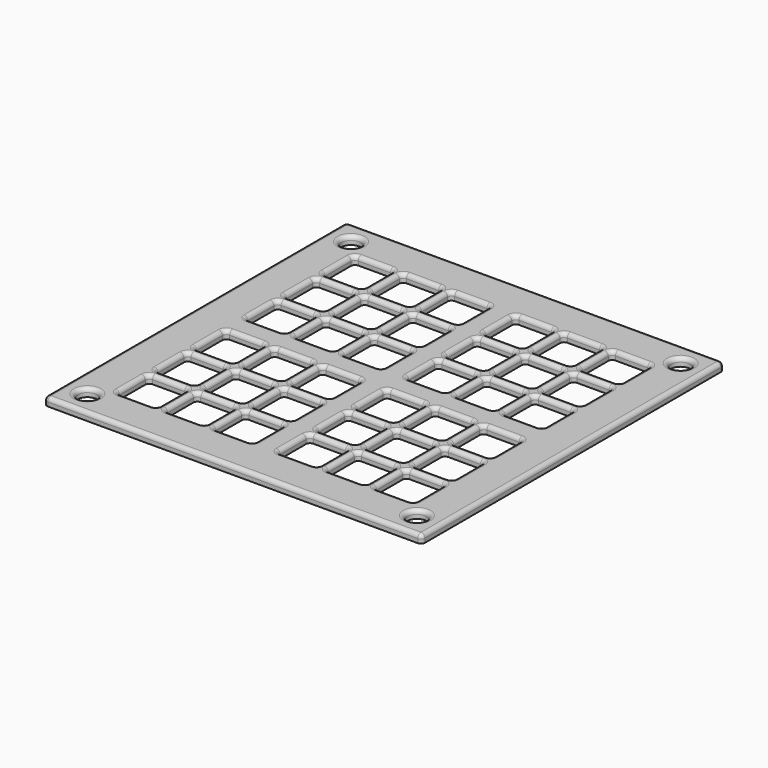
from build123d import *

# Parameters (mm, degrees)
F0_W     = 119.38
F0_H     = 119.38
F0_R     = 3.048
F1_DEPTH = 2.54
F2_R     = 1.26999


# Not quite as in the source:
# - a fillet or chamfer is up to 0.001 mm smaller than in the source, because OpenCascade refuses the exact size


with BuildPart() as f1:
    # F0 (on Top) → F1 (new body)
    with BuildSketch(Plane.XY):
        Rectangle(F0_W, F0_H)
        with Locations((-52.07, -52.07)):
            Circle(F0_R, mode=Mode.SUBTRACT)
        with BuildLine():
            Line((-46.99, -45.72), (-46.99, -35.56))
            ThreePointArc((-46.99, -35.56), (-46.6180256121, -34.6619743879), (-45.72, -34.29))
            Line((-45.72, -34.29), (-35.56, -34.29))
            ThreePointArc((-35.56, -34.29), (-34.6619743879, -34.6619743879), (-34.29, -35.56))
            Line((-34.29, -35.56), (-34.29, -45.72))
            ThreePointArc((-34.29, -45.72), (-34.6619743879, -46.6180256121), (-35.56, -46.99))
            Line((-35.56, -46.99), (-45.72, -46.99))
            ThreePointArc((-45.72, -46.99), (-46.6180256121, -46.6180256121), (-46.99, -45.72))
        make_face(mode=Mode.SUBTRACT)
        with BuildLine():
            Line((-20.32, -46.99), (-30.48, -46.99))
            ThreePointArc((-30.48, -46.99), (-31.3780256121, -46.6180256121), (-31.75, -45.72))
            Line((-31.75, -45.72), (-31.75, -35.56))
            ThreePointArc((-31.75, -35.56), (-31.3780256121, -34.6619743879), (-30.48, -34.29))
            Line((-30.48, -34.29), (-20.32, -34.29))
            ThreePointArc((-20.32, -34.29), (-19.4219743879, -34.6619743879), (-19.05, -35.56))
            Line((-19.05, -35.56), (-19.05, -45.72))
            ThreePointArc((-19.05, -45.72), (-19.4219743879, -46.6180256121), (-20.32, -46.99))
        make_face(mode=Mode.SUBTRACT)
        with BuildLine():
            Line((-15.24, -34.29), (-5.08, -34.29))
            ThreePointArc((-5.08, -34.29), (-4.1819743879, -34.6619743879), (-3.81, -35.56))
            Line((-3.81, -35.56), (-3.81, -45.72))
            ThreePointArc((-3.81, -45.72), (-4.1819743879, -46.6180256121), (-5.08, -46.99))
            Line((-5.08, -46.99), (-15.24, -46.99))
            ThreePointArc((-15.24, -46.99), (-16.1380256121, -46.6180256121), (-16.51, -45.72))
            Line((-16.51, -45.72), (-16.51, -35.56))
            ThreePointArc((-16.51, -35.56), (-16.1380256121, -34.6619743879), (-15.24, -34.29))
        make_face(mode=Mode.SUBTRACT)
        with BuildLine():
            Line((-34.29, -20.32), (-34.29, -30.48))
            ThreePointArc((-34.29, -30.48), (-34.6619743879, -31.3780256121), (-35.56, -31.75))
            Line((-35.56, -31.75), (-45.72, -31.75))
            ThreePointArc((-45.72, -31.75), (-46.6180256121, -31.3780256121), (-46.99, -30.48))
            Line((-46.99, -30.48), (-46.99, -20.32))
            ThreePointArc((-46.99, -20.32), (-46.6180256121, -19.4219743879), (-45.72, -19.05))
            Line((-45.72, -19.05), (-35.56, -19.05))
            ThreePointArc((-35.56, -19.05), (-34.6619743879, -19.4219743879), (-34.29, -20.32))
        make_face(mode=Mode.SUBTRACT)
        with BuildLine():
            Line((-45.72, -3.81), (-35.56, -3.81))
            ThreePointArc((-35.56, -3.81), (-34.6619743879, -4.1819743879), (-34.29, -5.08))
            Line((-34.29, -5.08), (-34.29, -15.24))
            ThreePointArc((-34.29, -15.24), (-34.6619743879, -16.1380256121), (-35.56, -16.51))
            Line((-35.56, -16.51), (-45.72, -16.51))
            ThreePointArc((-45.72, -16.51), (-46.6180256121, -16.1380256121), (-46.99, -15.24))
            Line((-46.99, -15.24), (-46.99, -5.08))
            ThreePointArc((-46.99, -5.08), (-46.6180256121, -4.1819743879), (-45.72, -3.81))
        make_face(mode=Mode.SUBTRACT)
        with BuildLine():
            Line((-30.48, -19.05), (-20.32, -19.05))
            ThreePointArc((-20.32, -19.05), (-19.4219743879, -19.4219743879), (-19.05, -20.32))
            Line((-19.05, -20.32), (-19.05, -30.48))
            ThreePointArc((-19.05, -30.48), (-19.4219743879, -31.3780256121), (-20.32, -31.75))
            Line((-20.32, -31.75), (-30.48, -31.75))
            ThreePointArc((-30.48, -31.75), (-31.3780256121, -31.3780256121), (-31.75, -30.48))
            Line((-31.75, -30.48), (-31.75, -20.32))
            ThreePointArc((-31.75, -20.32), (-31.3780256121, -19.4219743879), (-30.48, -19.05))
        make_face(mode=Mode.SUBTRACT)
        with BuildLine():
            Line((-5.08, -31.75), (-15.24, -31.75))
            ThreePointArc((-15.24, -31.75), (-16.1380256121, -31.3780256121), (-16.51, -30.48))
            Line((-16.51, -30.48), (-16.51, -20.32))
            ThreePointArc((-16.51, -20.32), (-16.1380256121, -19.4219743879), (-15.24, -19.05))
            Line((-15.24, -19.05), (-5.08, -19.05))
            ThreePointArc((-5.08, -19.05), (-4.1819743879, -19.4219743879), (-3.81, -20.32))
            Line((-3.81, -20.32), (-3.81, -30.48))
            ThreePointArc((-3.81, -30.48), (-4.1819743879, -31.3780256121), (-5.08, -31.75))
        make_face(mode=Mode.SUBTRACT)
        with BuildLine():
            Line((-31.75, -15.24), (-31.75, -5.08))
            ThreePointArc((-31.75, -5.08), (-31.3780256121, -4.1819743879), (-30.48, -3.81))
            Line((-30.48, -3.81), (-20.32, -3.81))
            ThreePointArc((-20.32, -3.81), (-19.4219743879, -4.1819743879), (-19.05, -5.08))
            Line((-19.05, -5.08), (-19.05, -15.24))
            ThreePointArc((-19.05, -15.24), (-19.4219743879, -16.1380256121), (-20.32, -16.51))
            Line((-20.32, -16.51), (-30.48, -16.51))
            ThreePointArc((-30.48, -16.51), (-31.3780256121, -16.1380256121), (-31.75, -15.24))
        make_face(mode=Mode.SUBTRACT)
        with BuildLine():
            Line((-15.24, -3.81), (-5.08, -3.81))
            ThreePointArc((-5.08, -3.81), (-4.1819743879, -4.1819743879), (-3.81, -5.08))
            Line((-3.81, -5.08), (-3.81, -15.24))
            ThreePointArc((-3.81, -15.24), (-4.1819743879, -16.1380256121), (-5.08, -16.51))
            Line((-5.08, -16.51), (-15.24, -16.51))
            ThreePointArc((-15.24, -16.51), (-16.1380256121, -16.1380256121), (-16.51, -15.24))
            Line((-16.51, -15.24), (-16.51, -5.08))
            ThreePointArc((-16.51, -5.08), (-16.1380256121, -4.1819743879), (-15.24, -3.81))
        make_face(mode=Mode.SUBTRACT)
        with BuildLine():
            Line((3.81, -45.72), (3.81, -35.56))
            ThreePointArc((3.81, -35.56), (4.1819743879, -34.6619743879), (5.08, -34.29))
            Line((5.08, -34.29), (15.24, -34.29))
            ThreePointArc((15.24, -34.29), (16.1380256121, -34.6619743879), (16.51, -35.56))
            Line((16.51, -35.56), (16.51, -45.72))
            ThreePointArc((16.51, -45.72), (16.1380256121, -46.6180256121), (15.24, -46.99))
            Line((15.24, -46.99), (5.08, -46.99))
            ThreePointArc((5.08, -46.99), (4.1819743879, -46.6180256121), (3.81, -45.72))
        make_face(mode=Mode.SUBTRACT)
        with BuildLine():
            Line((19.05, -45.72), (19.05, -35.56))
            ThreePointArc((19.05, -35.56), (19.4219743879, -34.6619743879), (20.32, -34.29))
            Line((20.32, -34.29), (30.48, -34.29))
            ThreePointArc((30.48, -34.29), (31.3780256121, -34.6619743879), (31.75, -35.56))
            Line((31.75, -35.56), (31.75, -45.72))
            ThreePointArc((31.75, -45.72), (31.3780256121, -46.6180256121), (30.48, -46.99))
            Line((30.48, -46.99), (20.32, -46.99))
            ThreePointArc((20.32, -46.99), (19.4219743879, -46.6180256121), (19.05, -45.72))
        make_face(mode=Mode.SUBTRACT)
        with Locations((52.07, -52.07)):
            Circle(F0_R, mode=Mode.SUBTRACT)
        with BuildLine():
            ThreePointArc((34.29, -35.56), (34.6619743879, -34.6619743879), (35.56, -34.29))
            Line((35.56, -34.29), (45.72, -34.29))
            ThreePointArc((45.72, -34.29), (46.6180256121, -34.6619743879), (46.99, -35.56))
            Line((46.99, -35.56), (46.99, -45.72))
            ThreePointArc((46.99, -45.72), (46.6180256121, -46.6180256121), (45.72, -46.99))
            Line((45.72, -46.99), (35.56, -46.99))
            ThreePointArc((35.56, -46.99), (34.6619743879, -46.6180256121), (34.29, -45.72))
            Line((34.29, -45.72), (34.29, -35.56))
        make_face(mode=Mode.SUBTRACT)
        with BuildLine():
            Line((3.81, -30.48), (3.81, -20.32))
            ThreePointArc((3.81, -20.32), (4.1819743879, -19.4219743879), (5.08, -19.05))
            Line((5.08, -19.05), (15.24, -19.05))
            ThreePointArc((15.24, -19.05), (16.1380256121, -19.4219743879), (16.51, -20.32))
            Line((16.51, -20.32), (16.51, -30.48))
            ThreePointArc((16.51, -30.48), (16.1380256121, -31.3780256121), (15.24, -31.75))
            Line((15.24, -31.75), (5.08, -31.75))
            ThreePointArc((5.08, -31.75), (4.1819743879, -31.3780256121), (3.81, -30.48))
        make_face(mode=Mode.SUBTRACT)
        with BuildLine():
            Line((19.05, -30.48), (19.05, -20.32))
            ThreePointArc((19.05, -20.32), (19.4219743879, -19.4219743879), (20.32, -19.05))
            Line((20.32, -19.05), (30.48, -19.05))
            ThreePointArc((30.48, -19.05), (31.3780256121, -19.4219743879), (31.75, -20.32))
            Line((31.75, -20.32), (31.75, -30.48))
            ThreePointArc((31.75, -30.48), (31.3780256121, -31.3780256121), (30.48, -31.75))
            Line((30.48, -31.75), (20.32, -31.75))
            ThreePointArc((20.32, -31.75), (19.4219743879, -31.3780256121), (19.05, -30.48))
        make_face(mode=Mode.SUBTRACT)
        with BuildLine():
            Line((3.81, -15.24), (3.81, -5.08))
            ThreePointArc((3.81, -5.08), (4.1819743879, -4.1819743879), (5.08, -3.81))
            Line((5.08, -3.81), (15.24, -3.81))
            ThreePointArc((15.24, -3.81), (16.1380256121, -4.1819743879), (16.51, -5.08))
            Line((16.51, -5.08), (16.51, -15.24))
            ThreePointArc((16.51, -15.24), (16.1380256121, -16.1380256121), (15.24, -16.51))
            Line((15.24, -16.51), (5.08, -16.51))
            ThreePointArc((5.08, -16.51), (4.1819743879, -16.1380256121), (3.81, -15.24))
        make_face(mode=Mode.SUBTRACT)
        with BuildLine():
            Line((19.05, -15.24), (19.05, -5.08))
            ThreePointArc((19.05, -5.08), (19.4219743879, -4.1819743879), (20.32, -3.81))
            Line((20.32, -3.81), (30.48, -3.81))
            ThreePointArc((30.48, -3.81), (31.3780256121, -4.1819743879), (31.75, -5.08))
            Line((31.75, -5.08), (31.75, -15.24))
            ThreePointArc((31.75, -15.24), (31.3780256121, -16.1380256121), (30.48, -16.51))
            Line((30.48, -16.51), (20.32, -16.51))
            ThreePointArc((20.32, -16.51), (19.4219743879, -16.1380256121), (19.05, -15.24))
        make_face(mode=Mode.SUBTRACT)
        with BuildLine():
            Line((34.29, -30.48), (34.29, -20.32))
            ThreePointArc((34.29, -20.32), (34.6619743879, -19.4219743879), (35.56, -19.05))
            Line((35.56, -19.05), (45.72, -19.05))
            ThreePointArc((45.72, -19.05), (46.6180256121, -19.4219743879), (46.99, -20.32))
            Line((46.99, -20.32), (46.99, -30.48))
            ThreePointArc((46.99, -30.48), (46.6180256121, -31.3780256121), (45.72, -31.75))
            Line((45.72, -31.75), (35.56, -31.75))
            ThreePointArc((35.56, -31.75), (34.6619743879, -31.3780256121), (34.29, -30.48))
        make_face(mode=Mode.SUBTRACT)
        with BuildLine():
            Line((34.29, -15.24), (34.29, -5.08))
            ThreePointArc((34.29, -5.08), (34.6619743879, -4.1819743879), (35.56, -3.81))
            Line((35.56, -3.81), (45.72, -3.81))
            ThreePointArc((45.72, -3.81), (46.6180256121, -4.1819743879), (46.99, -5.08))
            Line((46.99, -5.08), (46.99, -15.24))
            ThreePointArc((46.99, -15.24), (46.6180256121, -16.1380256121), (45.72, -16.51))
            Line((45.72, -16.51), (35.56, -16.51))
            ThreePointArc((35.56, -16.51), (34.6619743879, -16.1380256121), (34.29, -15.24))
        make_face(mode=Mode.SUBTRACT)
        with BuildLine():
            ThreePointArc((-46.99, 15.24), (-46.6180256121, 16.1380256121), (-45.72, 16.51))
            Line((-45.72, 16.51), (-35.56, 16.51))
            ThreePointArc((-35.56, 16.51), (-34.6619743879, 16.1380256121), (-34.29, 15.24))
            Line((-34.29, 15.24), (-34.29, 5.08))
            ThreePointArc((-34.29, 5.08), (-34.6619743879, 4.1819743879), (-35.56, 3.81))
            Line((-35.56, 3.81), (-45.72, 3.81))
            ThreePointArc((-45.72, 3.81), (-46.6180256121, 4.1819743879), (-46.99, 5.08))
            Line((-46.99, 5.08), (-46.99, 15.24))
        make_face(mode=Mode.SUBTRACT)
        with BuildLine():
            ThreePointArc((-34.29, 20.32), (-34.6619743879, 19.4219743879), (-35.56, 19.05))
            Line((-35.56, 19.05), (-45.72, 19.05))
            ThreePointArc((-45.72, 19.05), (-46.6180256121, 19.4219743879), (-46.99, 20.32))
            Line((-46.99, 20.32), (-46.99, 30.48))
            ThreePointArc((-46.99, 30.48), (-46.6180256121, 31.3780256121), (-45.72, 31.75))
            Line((-45.72, 31.75), (-35.56, 31.75))
            ThreePointArc((-35.56, 31.75), (-34.6619743879, 31.3780256121), (-34.29, 30.48))
            Line((-34.29, 30.48), (-34.29, 20.32))
        make_face(mode=Mode.SUBTRACT)
        with BuildLine():
            ThreePointArc((-30.48, 3.81), (-31.3780256121, 4.1819743879), (-31.75, 5.08))
            Line((-31.75, 5.08), (-31.75, 15.24))
            ThreePointArc((-31.75, 15.24), (-31.3780256121, 16.1380256121), (-30.48, 16.51))
            Line((-30.48, 16.51), (-20.32, 16.51))
            ThreePointArc((-20.32, 16.51), (-19.4219743879, 16.1380256121), (-19.05, 15.24))
            Line((-19.05, 15.24), (-19.05, 5.08))
            ThreePointArc((-19.05, 5.08), (-19.4219743879, 4.1819743879), (-20.32, 3.81))
            Line((-20.32, 3.81), (-30.48, 3.81))
        make_face(mode=Mode.SUBTRACT)
        with BuildLine():
            ThreePointArc((-15.24, 3.81), (-16.1380256121, 4.1819743879), (-16.51, 5.08))
            Line((-16.51, 5.08), (-16.51, 15.24))
            ThreePointArc((-16.51, 15.24), (-16.1380256121, 16.1380256121), (-15.24, 16.51))
            Line((-15.24, 16.51), (-5.08, 16.51))
            ThreePointArc((-5.08, 16.51), (-4.1819743879, 16.1380256121), (-3.81, 15.24))
            Line((-3.81, 15.24), (-3.81, 5.08))
            ThreePointArc((-3.81, 5.08), (-4.1819743879, 4.1819743879), (-5.08, 3.81))
            Line((-5.08, 3.81), (-15.24, 3.81))
        make_face(mode=Mode.SUBTRACT)
        with BuildLine():
            ThreePointArc((-31.75, 30.48), (-31.3780256121, 31.3780256121), (-30.48, 31.75))
            Line((-30.48, 31.75), (-20.32, 31.75))
            ThreePointArc((-20.32, 31.75), (-19.4219743879, 31.3780256121), (-19.05, 30.48))
            Line((-19.05, 30.48), (-19.05, 20.32))
            ThreePointArc((-19.05, 20.32), (-19.4219743879, 19.4219743879), (-20.32, 19.05))
            Line((-20.32, 19.05), (-30.48, 19.05))
            ThreePointArc((-30.48, 19.05), (-31.3780256121, 19.4219743879), (-31.75, 20.32))
            Line((-31.75, 20.32), (-31.75, 30.48))
        make_face(mode=Mode.SUBTRACT)
        with BuildLine():
            ThreePointArc((-15.24, 19.05), (-16.1380256121, 19.4219743879), (-16.51, 20.32))
            Line((-16.51, 20.32), (-16.51, 30.48))
            ThreePointArc((-16.51, 30.48), (-16.1380256121, 31.3780256121), (-15.24, 31.75))
            Line((-15.24, 31.75), (-5.08, 31.75))
            ThreePointArc((-5.08, 31.75), (-4.1819743879, 31.3780256121), (-3.81, 30.48))
            Line((-3.81, 30.48), (-3.81, 20.32))
            ThreePointArc((-3.81, 20.32), (-4.1819743879, 19.4219743879), (-5.08, 19.05))
            Line((-5.08, 19.05), (-15.24, 19.05))
        make_face(mode=Mode.SUBTRACT)
        with BuildLine():
            ThreePointArc((-35.56, 46.99), (-34.6619743879, 46.6180256121), (-34.29, 45.72))
            Line((-34.29, 45.72), (-34.29, 35.56))
            ThreePointArc((-34.29, 35.56), (-34.6619743879, 34.6619743879), (-35.56, 34.29))
            Line((-35.56, 34.29), (-45.72, 34.29))
            ThreePointArc((-45.72, 34.29), (-46.6180256121, 34.6619743879), (-46.99, 35.56))
            Line((-46.99, 35.56), (-46.99, 45.72))
            ThreePointArc((-46.99, 45.72), (-46.6180256121, 46.6180256121), (-45.72, 46.99))
            Line((-45.72, 46.99), (-35.56, 46.99))
        make_face(mode=Mode.SUBTRACT)
        with Locations((-52.07, 52.07)):
            Circle(F0_R, mode=Mode.SUBTRACT)
        with BuildLine():
            ThreePointArc((-31.75, 45.72), (-31.3780256121, 46.6180256121), (-30.48, 46.99))
            Line((-30.48, 46.99), (-20.32, 46.99))
            ThreePointArc((-20.32, 46.99), (-19.4219743879, 46.6180256121), (-19.05, 45.72))
            Line((-19.05, 45.72), (-19.05, 35.56))
            ThreePointArc((-19.05, 35.56), (-19.4219743879, 34.6619743879), (-20.32, 34.29))
            Line((-20.32, 34.29), (-30.48, 34.29))
            ThreePointArc((-30.48, 34.29), (-31.3780256121, 34.6619743879), (-31.75, 35.56))
            Line((-31.75, 35.56), (-31.75, 45.72))
        make_face(mode=Mode.SUBTRACT)
        with BuildLine():
            ThreePointArc((-16.51, 45.72), (-16.1380256121, 46.6180256121), (-15.24, 46.99))
            Line((-15.24, 46.99), (-5.08, 46.99))
            ThreePointArc((-5.08, 46.99), (-4.1819743879, 46.6180256121), (-3.81, 45.72))
            Line((-3.81, 45.72), (-3.81, 35.56))
            ThreePointArc((-3.81, 35.56), (-4.1819743879, 34.6619743879), (-5.08, 34.29))
            Line((-5.08, 34.29), (-15.24, 34.29))
            ThreePointArc((-15.24, 34.29), (-16.1380256121, 34.6619743879), (-16.51, 35.56))
            Line((-16.51, 35.56), (-16.51, 45.72))
        make_face(mode=Mode.SUBTRACT)
        with BuildLine():
            Line((15.24, 3.81), (5.08, 3.81))
            ThreePointArc((5.08, 3.81), (4.1819743879, 4.1819743879), (3.81, 5.08))
            Line((3.81, 5.08), (3.81, 15.24))
            ThreePointArc((3.81, 15.24), (4.1819743879, 16.1380256121), (5.08, 16.51))
            Line((5.08, 16.51), (15.24, 16.51))
            ThreePointArc((15.24, 16.51), (16.1380256121, 16.1380256121), (16.51, 15.24))
            Line((16.51, 15.24), (16.51, 5.08))
            ThreePointArc((16.51, 5.08), (16.1380256121, 4.1819743879), (15.24, 3.81))
        make_face(mode=Mode.SUBTRACT)
        with BuildLine():
            Line((19.05, 5.08), (19.05, 15.24))
            ThreePointArc((19.05, 15.24), (19.4219743879, 16.1380256121), (20.32, 16.51))
            Line((20.32, 16.51), (30.48, 16.51))
            ThreePointArc((30.48, 16.51), (31.3780256121, 16.1380256121), (31.75, 15.24))
            Line((31.75, 15.24), (31.75, 5.08))
            ThreePointArc((31.75, 5.08), (31.3780256121, 4.1819743879), (30.48, 3.81))
            Line((30.48, 3.81), (20.32, 3.81))
            ThreePointArc((20.32, 3.81), (19.4219743879, 4.1819743879), (19.05, 5.08))
        make_face(mode=Mode.SUBTRACT)
        with BuildLine():
            Line((3.81, 20.32), (3.81, 30.48))
            ThreePointArc((3.81, 30.48), (4.1819743879, 31.3780256121), (5.08, 31.75))
            Line((5.08, 31.75), (15.24, 31.75))
            ThreePointArc((15.24, 31.75), (16.1380256121, 31.3780256121), (16.51, 30.48))
            Line((16.51, 30.48), (16.51, 20.32))
            ThreePointArc((16.51, 20.32), (16.1380256121, 19.4219743879), (15.24, 19.05))
            Line((15.24, 19.05), (5.08, 19.05))
            ThreePointArc((5.08, 19.05), (4.1819743879, 19.4219743879), (3.81, 20.32))
        make_face(mode=Mode.SUBTRACT)
        with BuildLine():
            Line((30.48, 19.05), (20.32, 19.05))
            ThreePointArc((20.32, 19.05), (19.4219743879, 19.4219743879), (19.05, 20.32))
            Line((19.05, 20.32), (19.05, 30.48))
            ThreePointArc((19.05, 30.48), (19.4219743879, 31.3780256121), (20.32, 31.75))
            Line((20.32, 31.75), (30.48, 31.75))
            ThreePointArc((30.48, 31.75), (31.3780256121, 31.3780256121), (31.75, 30.48))
            Line((31.75, 30.48), (31.75, 20.32))
            ThreePointArc((31.75, 20.32), (31.3780256121, 19.4219743879), (30.48, 19.05))
        make_face(mode=Mode.SUBTRACT)
        with BuildLine():
            Line((45.72, 3.81), (35.56, 3.81))
            ThreePointArc((35.56, 3.81), (34.6619743879, 4.1819743879), (34.29, 5.08))
            Line((34.29, 5.08), (34.29, 15.24))
            ThreePointArc((34.29, 15.24), (34.6619743879, 16.1380256121), (35.56, 16.51))
            Line((35.56, 16.51), (45.72, 16.51))
            ThreePointArc((45.72, 16.51), (46.6180256121, 16.1380256121), (46.99, 15.24))
            Line((46.99, 15.24), (46.99, 5.08))
            ThreePointArc((46.99, 5.08), (46.6180256121, 4.1819743879), (45.72, 3.81))
        make_face(mode=Mode.SUBTRACT)
        with BuildLine():
            Line((35.56, 31.75), (45.72, 31.75))
            ThreePointArc((45.72, 31.75), (46.6180256121, 31.3780256121), (46.99, 30.48))
            Line((46.99, 30.48), (46.99, 20.32))
            ThreePointArc((46.99, 20.32), (46.6180256121, 19.4219743879), (45.72, 19.05))
            Line((45.72, 19.05), (35.56, 19.05))
            ThreePointArc((35.56, 19.05), (34.6619743879, 19.4219743879), (34.29, 20.32))
            Line((34.29, 20.32), (34.29, 30.48))
            ThreePointArc((34.29, 30.48), (34.6619743879, 31.3780256121), (35.56, 31.75))
        make_face(mode=Mode.SUBTRACT)
        with BuildLine():
            Line((15.24, 34.29), (5.08, 34.29))
            ThreePointArc((5.08, 34.29), (4.1819743879, 34.6619743879), (3.81, 35.56))
            Line((3.81, 35.56), (3.81, 45.72))
            ThreePointArc((3.81, 45.72), (4.1819743879, 46.6180256121), (5.08, 46.99))
            Line((5.08, 46.99), (15.24, 46.99))
            ThreePointArc((15.24, 46.99), (16.1380256121, 46.6180256121), (16.51, 45.72))
            Line((16.51, 45.72), (16.51, 35.56))
            ThreePointArc((16.51, 35.56), (16.1380256121, 34.6619743879), (15.24, 34.29))
        make_face(mode=Mode.SUBTRACT)
        with BuildLine():
            Line((19.05, 35.56), (19.05, 45.72))
            ThreePointArc((19.05, 45.72), (19.4219743879, 46.6180256121), (20.32, 46.99))
            Line((20.32, 46.99), (30.48, 46.99))
            ThreePointArc((30.48, 46.99), (31.3780256121, 46.6180256121), (31.75, 45.72))
            Line((31.75, 45.72), (31.75, 35.56))
            ThreePointArc((31.75, 35.56), (31.3780256121, 34.6619743879), (30.48, 34.29))
            Line((30.48, 34.29), (20.32, 34.29))
            ThreePointArc((20.32, 34.29), (19.4219743879, 34.6619743879), (19.05, 35.56))
        make_face(mode=Mode.SUBTRACT)
        with BuildLine():
            Line((35.56, 46.99), (45.72, 46.99))
            ThreePointArc((45.72, 46.99), (46.6180256121, 46.6180256121), (46.99, 45.72))
            Line((46.99, 45.72), (46.99, 35.56))
            ThreePointArc((46.99, 35.56), (46.6180256121, 34.6619743879), (45.72, 34.29))
            Line((45.72, 34.29), (35.56, 34.29))
            ThreePointArc((35.56, 34.29), (34.6619743879, 34.6619743879), (34.29, 35.56))
            Line((34.29, 35.56), (34.29, 45.72))
            ThreePointArc((34.29, 45.72), (34.6619743879, 46.6180256121), (35.56, 46.99))
        make_face(mode=Mode.SUBTRACT)
        with Locations((52.07, 52.07)):
            Circle(F0_R, mode=Mode.SUBTRACT)
    extrude(amount=F1_DEPTH)

    # F2 (radius 1.27 in the source; OpenCascade refuses exactly that, so slightly less here)
    f2_edges = [f1.edges().sort_by_distance(p)[0] for p in [
        (0, -59.69, 2.54),
        (59.69, 0, 2.54),
        (0, 59.69, 2.54),
        (-59.69, 0, 2.54),
        (-55.118, -52.07, 2.54),
        (-46.99, -40.64, 2.54),
        (-46.618026, -34.661974, 2.54),
        (-40.64, -34.29, 2.54),
        (-34.661974, -34.661974, 2.54),
        (-34.29, -40.64, 2.54),
        (-34.661974, -46.618026, 2.54),
        (-40.64, -46.99, 2.54),
        (-46.618026, -46.618026, 2.54),
        (-19.421974, -46.618026, 2.54),
        (-25.4, -46.99, 2.54),
        (-31.378026, -46.618026, 2.54),
        (-31.75, -40.64, 2.54),
        (-31.378026, -34.661974, 2.54),
        (-25.4, -34.29, 2.54),
        (-19.421974, -34.661974, 2.54),
        (-19.05, -40.64, 2.54),
        (-10.16, -34.29, 2.54),
        (-4.181974, -34.661974, 2.54),
        (-3.81, -40.64, 2.54),
        (-4.181974, -46.618026, 2.54),
        (-10.16, -46.99, 2.54),
        (-16.138026, -46.618026, 2.54),
        (-16.51, -40.64, 2.54),
        (-16.138026, -34.661974, 2.54),
        (-34.29, -25.4, 2.54),
        (-34.661974, -31.378026, 2.54),
        (-40.64, -31.75, 2.54),
        (-46.618026, -31.378026, 2.54),
        (-46.99, -25.4, 2.54),
        (-46.618026, -19.421974, 2.54),
        (-40.64, -19.05, 2.54),
        (-34.661974, -19.421974, 2.54),
        (-40.64, -3.81, 2.54),
        (-34.661974, -4.181974, 2.54),
        (-34.29, -10.16, 2.54),
        (-34.661974, -16.138026, 2.54),
        (-40.64, -16.51, 2.54),
        (-46.618026, -16.138026, 2.54),
        (-46.99, -10.16, 2.54),
        (-46.618026, -4.181974, 2.54),
        (-25.4, -19.05, 2.54),
        (-19.421974, -19.421974, 2.54),
        (-19.05, -25.4, 2.54),
        (-19.421974, -31.378026, 2.54),
        (-25.4, -31.75, 2.54),
        (-31.378026, -31.378026, 2.54),
        (-31.75, -25.4, 2.54),
        (-31.378026, -19.421974, 2.54),
        (-4.181974, -31.378026, 2.54),
        (-10.16, -31.75, 2.54),
        (-16.138026, -31.378026, 2.54),
        (-16.51, -25.4, 2.54),
        (-16.138026, -19.421974, 2.54),
        (-10.16, -19.05, 2.54),
        (-4.181974, -19.421974, 2.54),
        (-3.81, -25.4, 2.54),
        (-31.75, -10.16, 2.54),
        (-31.378026, -4.181974, 2.54),
        (-25.4, -3.81, 2.54),
        (-19.421974, -4.181974, 2.54),
        (-19.05, -10.16, 2.54),
        (-19.421974, -16.138026, 2.54),
        (-25.4, -16.51, 2.54),
        (-31.378026, -16.138026, 2.54),
        (-10.16, -3.81, 2.54),
        (-4.181974, -4.181974, 2.54),
        (-3.81, -10.16, 2.54),
        (-4.181974, -16.138026, 2.54),
        (-10.16, -16.51, 2.54),
        (-16.138026, -16.138026, 2.54),
        (-16.51, -10.16, 2.54),
        (-16.138026, -4.181974, 2.54),
        (3.81, -40.64, 2.54),
        (4.181974, -34.661974, 2.54),
        (10.16, -34.29, 2.54),
        (16.138026, -34.661974, 2.54),
        (16.51, -40.64, 2.54),
        (16.138026, -46.618026, 2.54),
        (10.16, -46.99, 2.54),
        (4.181974, -46.618026, 2.54),
        (19.05, -40.64, 2.54),
        (19.421974, -34.661974, 2.54),
        (25.4, -34.29, 2.54),
        (31.378026, -34.661974, 2.54),
        (31.75, -40.64, 2.54),
        (31.378026, -46.618026, 2.54),
        (25.4, -46.99, 2.54),
        (19.421974, -46.618026, 2.54),
        (49.022, -52.07, 2.54),
        (34.661974, -34.661974, 2.54),
        (40.64, -34.29, 2.54),
        (46.618026, -34.661974, 2.54),
        (46.99, -40.64, 2.54),
        (46.618026, -46.618026, 2.54),
        (40.64, -46.99, 2.54),
        (34.661974, -46.618026, 2.54),
        (34.29, -40.64, 2.54),
        (3.81, -25.4, 2.54),
        (4.181974, -19.421974, 2.54),
        (10.16, -19.05, 2.54),
        (16.138026, -19.421974, 2.54),
        (16.51, -25.4, 2.54),
        (16.138026, -31.378026, 2.54),
        (10.16, -31.75, 2.54),
        (4.181974, -31.378026, 2.54),
        (19.421974, -31.378026, 2.54),
        (19.05, -25.4, 2.54),
        (19.421974, -19.421974, 2.54),
        (25.4, -19.05, 2.54),
        (31.378026, -19.421974, 2.54),
        (31.75, -25.4, 2.54),
        (31.378026, -31.378026, 2.54),
        (25.4, -31.75, 2.54),
        (3.81, -10.16, 2.54),
        (4.181974, -4.181974, 2.54),
        (10.16, -3.81, 2.54),
        (16.138026, -4.181974, 2.54),
        (16.51, -10.16, 2.54),
        (16.138026, -16.138026, 2.54),
        (10.16, -16.51, 2.54),
        (4.181974, -16.138026, 2.54),
        (19.05, -10.16, 2.54),
        (19.421974, -4.181974, 2.54),
        (25.4, -3.81, 2.54),
        (31.378026, -4.181974, 2.54),
        (31.75, -10.16, 2.54),
        (31.378026, -16.138026, 2.54),
        (25.4, -16.51, 2.54),
        (19.421974, -16.138026, 2.54),
        (40.64, -31.75, 2.54),
        (34.661974, -31.378026, 2.54),
        (34.29, -25.4, 2.54),
        (34.661974, -19.421974, 2.54),
        (40.64, -19.05, 2.54),
        (46.618026, -19.421974, 2.54),
        (46.99, -25.4, 2.54),
        (46.618026, -31.378026, 2.54),
        (34.29, -10.16, 2.54),
        (34.661974, -4.181974, 2.54),
        (40.64, -3.81, 2.54),
        (46.618026, -4.181974, 2.54),
        (46.99, -10.16, 2.54),
        (46.618026, -16.138026, 2.54),
        (40.64, -16.51, 2.54),
        (34.661974, -16.138026, 2.54),
        (-46.618026, 4.181974, 2.54),
        (-46.99, 10.16, 2.54),
        (-46.618026, 16.138026, 2.54),
        (-40.64, 16.51, 2.54),
        (-34.661974, 16.138026, 2.54),
        (-34.29, 10.16, 2.54),
        (-34.661974, 4.181974, 2.54),
        (-40.64, 3.81, 2.54),
        (-34.661974, 31.378026, 2.54),
        (-34.29, 25.4, 2.54),
        (-34.661974, 19.421974, 2.54),
        (-40.64, 19.05, 2.54),
        (-46.618026, 19.421974, 2.54),
        (-46.99, 25.4, 2.54),
        (-46.618026, 31.378026, 2.54),
        (-40.64, 31.75, 2.54),
        (-31.378026, 4.181974, 2.54),
        (-31.75, 10.16, 2.54),
        (-31.378026, 16.138026, 2.54),
        (-25.4, 16.51, 2.54),
        (-19.421974, 16.138026, 2.54),
        (-19.05, 10.16, 2.54),
        (-19.421974, 4.181974, 2.54),
        (-25.4, 3.81, 2.54),
        (-16.138026, 4.181974, 2.54),
        (-16.51, 10.16, 2.54),
        (-16.138026, 16.138026, 2.54),
        (-10.16, 16.51, 2.54),
        (-4.181974, 16.138026, 2.54),
        (-3.81, 10.16, 2.54),
        (-4.181974, 4.181974, 2.54),
        (-10.16, 3.81, 2.54),
        (-31.378026, 31.378026, 2.54),
        (-25.4, 31.75, 2.54),
        (-19.421974, 31.378026, 2.54),
        (-19.05, 25.4, 2.54),
        (-19.421974, 19.421974, 2.54),
        (-25.4, 19.05, 2.54),
        (-31.378026, 19.421974, 2.54),
        (-31.75, 25.4, 2.54),
        (-16.138026, 19.421974, 2.54),
        (-16.51, 25.4, 2.54),
        (-16.138026, 31.378026, 2.54),
        (-10.16, 31.75, 2.54),
        (-4.181974, 31.378026, 2.54),
        (-3.81, 25.4, 2.54),
        (-4.181974, 19.421974, 2.54),
        (-10.16, 19.05, 2.54),
        (-40.64, 46.99, 2.54),
        (-34.661974, 46.618026, 2.54),
        (-34.29, 40.64, 2.54),
        (-34.661974, 34.661974, 2.54),
        (-40.64, 34.29, 2.54),
        (-46.618026, 34.661974, 2.54),
        (-46.99, 40.64, 2.54),
        (-46.618026, 46.618026, 2.54),
        (-55.118, 52.07, 2.54),
        (-31.378026, 46.618026, 2.54),
        (-25.4, 46.99, 2.54),
        (-19.421974, 46.618026, 2.54),
        (-19.05, 40.64, 2.54),
        (-19.421974, 34.661974, 2.54),
        (-25.4, 34.29, 2.54),
        (-31.378026, 34.661974, 2.54),
        (-31.75, 40.64, 2.54),
        (-16.51, 40.64, 2.54),
        (-16.138026, 46.618026, 2.54),
        (-10.16, 46.99, 2.54),
        (-4.181974, 46.618026, 2.54),
        (-3.81, 40.64, 2.54),
        (-4.181974, 34.661974, 2.54),
        (-10.16, 34.29, 2.54),
        (-16.138026, 34.661974, 2.54),
        (10.16, 3.81, 2.54),
        (4.181974, 4.181974, 2.54),
        (3.81, 10.16, 2.54),
        (4.181974, 16.138026, 2.54),
        (10.16, 16.51, 2.54),
        (16.138026, 16.138026, 2.54),
        (16.51, 10.16, 2.54),
        (16.138026, 4.181974, 2.54),
        (25.4, 3.81, 2.54),
        (19.421974, 4.181974, 2.54),
        (19.05, 10.16, 2.54),
        (19.421974, 16.138026, 2.54),
        (25.4, 16.51, 2.54),
        (31.378026, 16.138026, 2.54),
        (31.75, 10.16, 2.54),
        (31.378026, 4.181974, 2.54),
        (3.81, 25.4, 2.54),
        (4.181974, 31.378026, 2.54),
        (10.16, 31.75, 2.54),
        (16.138026, 31.378026, 2.54),
        (16.51, 25.4, 2.54),
        (16.138026, 19.421974, 2.54),
        (10.16, 19.05, 2.54),
        (4.181974, 19.421974, 2.54),
        (25.4, 19.05, 2.54),
        (19.421974, 19.421974, 2.54),
        (19.05, 25.4, 2.54),
        (19.421974, 31.378026, 2.54),
        (25.4, 31.75, 2.54),
        (31.378026, 31.378026, 2.54),
        (31.75, 25.4, 2.54),
        (31.378026, 19.421974, 2.54),
        (40.64, 3.81, 2.54),
        (34.661974, 4.181974, 2.54),
        (34.29, 10.16, 2.54),
        (34.661974, 16.138026, 2.54),
        (40.64, 16.51, 2.54),
        (46.618026, 16.138026, 2.54),
        (46.99, 10.16, 2.54),
        (46.618026, 4.181974, 2.54),
        (40.64, 31.75, 2.54),
        (46.618026, 31.378026, 2.54),
        (46.99, 25.4, 2.54),
        (46.618026, 19.421974, 2.54),
        (40.64, 19.05, 2.54),
        (34.661974, 19.421974, 2.54),
        (34.29, 25.4, 2.54),
        (34.661974, 31.378026, 2.54),
        (16.138026, 34.661974, 2.54),
        (10.16, 34.29, 2.54),
        (4.181974, 34.661974, 2.54),
        (3.81, 40.64, 2.54),
        (4.181974, 46.618026, 2.54),
        (10.16, 46.99, 2.54),
        (16.138026, 46.618026, 2.54),
        (16.51, 40.64, 2.54),
        (19.05, 40.64, 2.54),
        (19.421974, 46.618026, 2.54),
        (25.4, 46.99, 2.54),
        (31.378026, 46.618026, 2.54),
        (31.75, 40.64, 2.54),
        (31.378026, 34.661974, 2.54),
        (25.4, 34.29, 2.54),
        (19.421974, 34.661974, 2.54),
        (34.661974, 46.618026, 2.54),
        (40.64, 46.99, 2.54),
        (46.618026, 46.618026, 2.54),
        (46.99, 40.64, 2.54),
        (46.618026, 34.661974, 2.54),
        (40.64, 34.29, 2.54),
        (34.661974, 34.661974, 2.54),
        (34.29, 40.64, 2.54),
        (49.022, 52.07, 2.54),
        (59.69, 59.69, 1.27),
        (-59.69, 59.69, 1.27),
        (-59.69, -59.69, 1.27),
        (59.69, -59.69, 1.27),
    ]]
    fillet(f2_edges, radius=F2_R)


solid = f1.part
